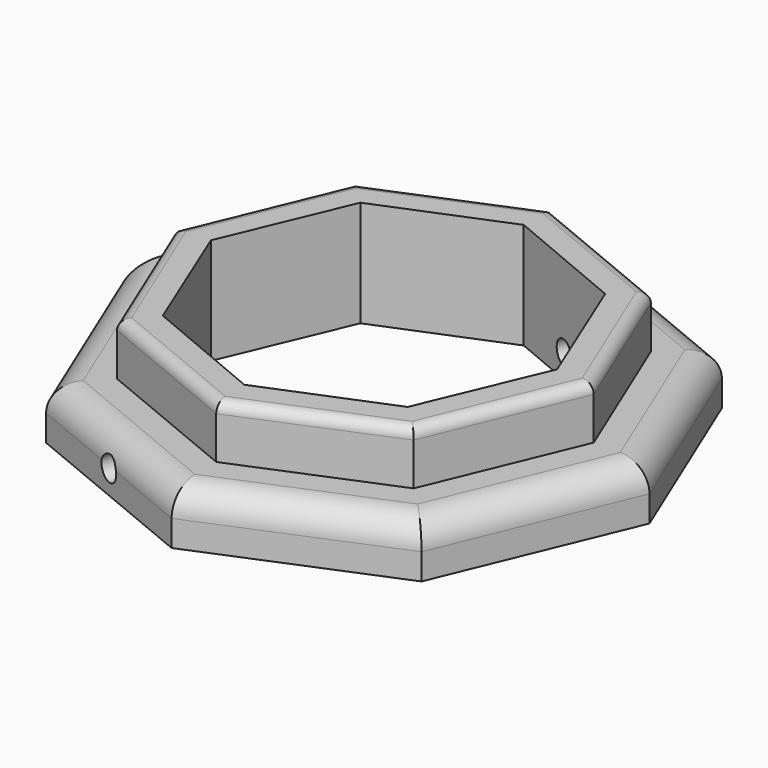
from build123d import *

# Parameters (mm, degrees)
F1_DEPTH     = 10
F3_DEPTH     = 10
F5_DEPTH     = 23.6474
F6_R         = 2.25
F7_DEPTH     = 107.696
F8_R         = 2
F9_T1_DEPTH  = 63.6683432365
F9_T3_DEPTH  = 63.6683432365
F9_T5_DEPTH  = 63.6683432365
F9_T7_DEPTH  = 63.6683432365
F9_T9_DEPTH  = 63.6683432365
F9_T11_DEPTH = 63.6683432365


# Not quite as in the source:
# - a fillet or chamfer that OpenCascade refuses, or shapes differently, is made with other operations: its cross-section is extruded or revolved along the edge and cut away or added


with BuildPart() as f1:
    # F0 (on Top) → F1 (new body)
    with BuildSketch(Plane.XY):
        Polygon((50, 0), (35.3553390593, 35.3553390593), (0, 50), (-35.3553390593, 35.3553390593), (-50, 0), (-35.3553390593, -35.3553390593), (0, -50), (35.3553390593, -35.3553390593), align=None)
    extrude(amount=-F1_DEPTH)

    # F2 (on face) → F3 (join)
    with BuildSketch(Plane.XY):
        Polygon((-27.9307178569, -27.9307178569), (0, -39.5), (27.9307178569, -27.9307178569), (39.5, 0), (27.9307178569, 27.9307178569), (0, 39.5), (-27.9307178569, 27.9307178569), (-39.5, 0), align=None)
    extrude(amount=F3_DEPTH)

    # F4 (on face) → F5 (cut)
    with BuildSketch(Plane.XY.offset(10)):
        Polygon((-32.7123950097, 0.1427250341), (-23.2320781797, -23.0302345008), (-0.1427250341, -32.7123950097), (23.0302345008, -23.2320781797), (32.7123950097, -0.1427250341), (23.2320781797, 23.0302345008), (0.1427250341, 32.7123950097), (-23.0302345008, 23.2320781797), align=None)
    extrude(amount=-F5_DEPTH, mode=Mode.SUBTRACT)

    # F6 (on face) → F7 (cut)
    with BuildSketch(Plane(origin=(17.6776695297, 42.6776695297, 0), x_dir=(-0.9238795325, 0.3826834324, 0), z_dir=(0.3826834324, 0.9238795325, 0))):
        with Locations((0, -5.5711902678)):
            Circle(F6_R)
    extrude(amount=-F7_DEPTH, mode=Mode.SUBTRACT)

    # F8
    f8_edges = [f1.edges().sort_by_distance(p)[0] for p in [
        (33.715359, 13.965359, 10),
        (33.715359, -13.965359, 10),
        (13.965359, -33.715359, 10),
        (-13.965359, -33.715359, 10),
        (-33.715359, -13.965359, 10),
        (-33.715359, 13.965359, 10),
        (-13.965359, 33.715359, 10),
        (13.965359, 33.715359, 10),
    ]]
    fillet(f8_edges, radius=F8_R)

    # F9: fillet of radius 5.08 on 6 edges, made by hand

    # F9_s2 → F9_t1 (cut)
    with BuildSketch(Plane(origin=(-12.1824100614, -29.4109395926, 0), x_dir=(0, 0, 1), z_dir=(0.3826834324, 0.9238795325, 0))):
        with BuildLine():
            ThreePointArc((0, 41.1139766256), (-1.4878975516, 44.706079074), (-5.08, 46.1939766256))
            Line((-5.08, 46.1939766256), (0, 46.1939766256))
            Line((0, 46.1939766256), (0, 41.1139766256))
        make_face()
    extrude(amount=F9_T1_DEPTH, mode=Mode.SUBTRACT)

    # F9_s4 → F9_t3 (cut)
    with BuildSketch(Plane(origin=(-29.4109395926, -12.1824100614, 0), x_dir=(0, 0, 1), z_dir=(0.9238795325, 0.3826834324, 0))):
        with BuildLine():
            ThreePointArc((0, 41.1139766256), (-1.4878975516, 44.706079074), (-5.08, 46.1939766256))
            Line((-5.08, 46.1939766256), (0, 46.1939766256))
            Line((0, 46.1939766256), (0, 41.1139766256))
        make_face()
    extrude(amount=F9_T3_DEPTH, mode=Mode.SUBTRACT)

    # F9_s6 → F9_t5 (cut)
    with BuildSketch(Plane(origin=(-29.4109395926, 12.1824100614, 0), x_dir=(0, 0, 1), z_dir=(0.9238795325, -0.3826834324, 0))):
        with BuildLine():
            ThreePointArc((0, 41.1139766256), (-1.4878975516, 44.706079074), (-5.08, 46.1939766256))
            Line((-5.08, 46.1939766256), (0, 46.1939766256))
            Line((0, 46.1939766256), (0, 41.1139766256))
        make_face()
    extrude(amount=F9_T5_DEPTH, mode=Mode.SUBTRACT)

    # F9_s8 → F9_t7 (cut)
    with BuildSketch(Plane(origin=(12.1824100614, -29.4109395926, 0), x_dir=(0, 0, 1), z_dir=(-0.3826834324, 0.9238795325, 0))):
        with BuildLine():
            ThreePointArc((0, 41.1139766256), (-1.4878975516, 44.706079074), (-5.08, 46.1939766256))
            Line((-5.08, 46.1939766256), (0, 46.1939766256))
            Line((0, 46.1939766256), (0, 41.1139766256))
        make_face()
    extrude(amount=F9_T7_DEPTH, mode=Mode.SUBTRACT)

    # F9_s10 → F9_t9 (cut)
    with BuildSketch(Plane(origin=(-12.1824100614, 29.4109395926, 0), x_dir=(0, 0, 1), z_dir=(0.3826834324, -0.9238795325, 0))):
        with BuildLine():
            ThreePointArc((0, 41.1139766256), (-1.4878975516, 44.706079074), (-5.08, 46.1939766256))
            Line((-5.08, 46.1939766256), (0, 46.1939766256))
            Line((0, 46.1939766256), (0, 41.1139766256))
        make_face()
    extrude(amount=F9_T9_DEPTH, mode=Mode.SUBTRACT)

    # F9_s12 → F9_t11 (cut)
    with BuildSketch(Plane(origin=(29.4109395926, -12.1824100614, 0), x_dir=(0, 0, 1), z_dir=(-0.9238795325, 0.3826834324, 0))):
        with BuildLine():
            ThreePointArc((0, 41.1139766256), (-1.4878975516, 44.706079074), (-5.08, 46.1939766256))
            Line((-5.08, 46.1939766256), (0, 46.1939766256))
            Line((0, 46.1939766256), (0, 41.1139766256))
        make_face()
    extrude(amount=F9_T11_DEPTH, mode=Mode.SUBTRACT)


solid = f1.part
